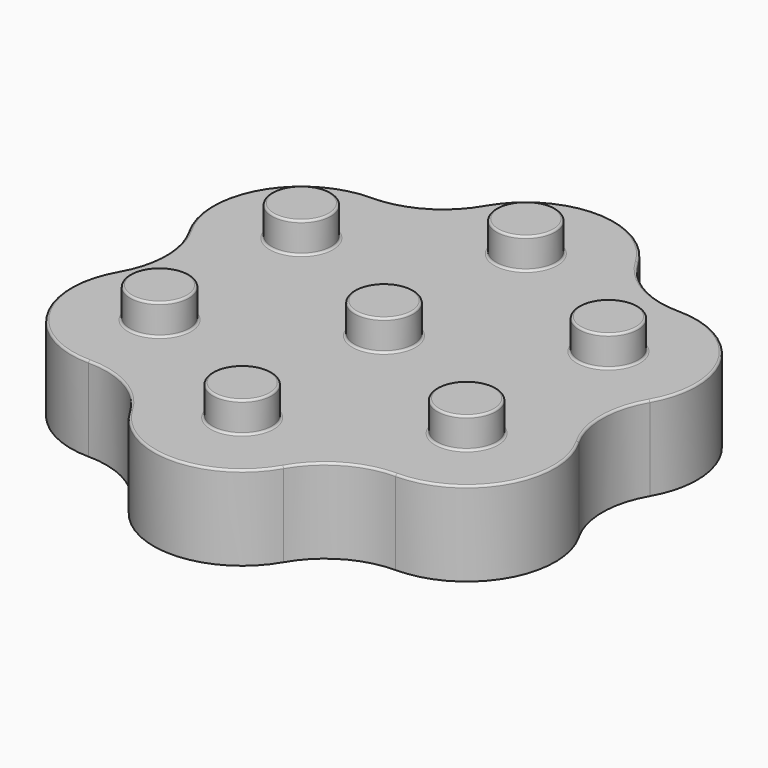
from build123d import *

# Parameters (mm, degrees)
F4_R     = 7.9
F5_DEPTH = 20
F6_DEPTH = 10
F7_R     = 7
F8_DEPTH = 7.3
F9_R     = 0.5


# Not quite as in the source:
# - a feature names something its author has since deleted; it is built from what else it names


with BuildPart() as f5:
    # F4 (on Top) → F5 (new body)
    with BuildSketch(Plane.XY):
        with BuildLine():
            ThreePointArc((18.1865334795, 10.5), (15.3730669589, 21), (18.1865334795, 31.5))
            ThreePointArc((18.1865334795, 31.5), (18.1865334795, 52.5), (0, 63))
            ThreePointArc((0, 63), (-10.5, 65.8134665205), (-18.1865334795, 73.5))
            ThreePointArc((-18.1865334795, 73.5), (-36.3730669589, 84), (-54.5596004384, 73.5))
            ThreePointArc((-54.5596004384, 73.5), (-62.2461339179, 65.8134665205), (-72.7461339179, 63))
            ThreePointArc((-72.7461339179, 63), (-90.9326673974, 52.5), (-90.9326673974, 31.5))
            ThreePointArc((-90.9326673974, 31.5), (-88.1192008768, 21), (-90.9326673974, 10.5))
            ThreePointArc((-90.9326673974, 10.5), (-90.9326673974, -10.5), (-72.7461339179, -21))
            ThreePointArc((-72.7461339179, -21), (-62.2461339179, -23.8134665205), (-54.5596004384, -31.5))
            ThreePointArc((-54.5596004384, -31.5), (-36.3730669589, -42), (-18.1865334795, -31.5))
            ThreePointArc((-18.1865334795, -31.5), (-10.5, -23.8134665205), (0, -21))
            ThreePointArc((0, -21), (18.1865334795, -10.5), (18.1865334795, 10.5))
        make_face()
        with Locations((-72.7461339179, 0)):
            Circle(F4_R, mode=Mode.SUBTRACT)
        with Locations((-36.3730669589, -21)):
            Circle(F4_R, mode=Mode.SUBTRACT)
        Circle(F4_R, mode=Mode.SUBTRACT)
        with Locations((-72.7461339179, 42)):
            Circle(F4_R, mode=Mode.SUBTRACT)
        with Locations((-36.3730669589, 21)):
            Circle(F4_R, mode=Mode.SUBTRACT)
        with Locations((0, 42)):
            Circle(F4_R, mode=Mode.SUBTRACT)
        with Locations((-36.3730669589, 63)):
            Circle(F4_R, mode=Mode.SUBTRACT)
        with Locations((0, 42)):
            Circle(F4_R)
        Circle(F4_R)
        with Locations((-36.3730669589, 21)):
            Circle(F4_R)
        with Locations((-36.3730669589, 63)):
            Circle(F4_R)
        with Locations((-72.7461339179, 42)):
            Circle(F4_R)
        with Locations((-72.7461339179, 0)):
            Circle(F4_R)
        with Locations((-36.3730669589, -21)):
            Circle(F4_R)
    extrude(amount=F5_DEPTH)

    # F4 (on Top) → F6 (cut)
    with BuildSketch(Plane.XY):
        with Locations((0, 42)):
            Circle(F4_R)
        Circle(F4_R)
        with Locations((-36.3730669589, 21)):
            Circle(F4_R)
        with Locations((-36.3730669589, 63)):
            Circle(F4_R)
        with Locations((-72.7461339179, 42)):
            Circle(F4_R)
        with Locations((-72.7461339179, 0)):
            Circle(F4_R)
        with Locations((-36.3730669589, -21)):
            Circle(F4_R)
    extrude(amount=F6_DEPTH, mode=Mode.SUBTRACT)

    # F7 (on face) → F8 (join)
    with BuildSketch(Plane.XY.offset(20)):
        Circle(F7_R)
        with Locations((0, 42)):
            Circle(F7_R)
        with Locations((-36.3730669589, 21)):
            Circle(F7_R)
        with Locations((-36.3730669589, 63)):
            Circle(F7_R)
        with Locations((-36.3730669589, -21)):
            Circle(F7_R)
        with Locations((-72.7461339179, 0)):
            Circle(F7_R)
        with Locations((-72.7461339179, 42)):
            Circle(F7_R)
    extrude(amount=F8_DEPTH)

    # F9
    f9_edges = [f5.edges().sort_by_distance(p)[0] for p in [
        (-7, 0, 27.3),
        (-7.9, 42, 0),
        (-7.9, 42, 10),
        (-7.9, 0, 0),
        (-7.9, 0, 10),
        (-7, 42, 27.3),
        (-7, 42, 20),
        (18.186533, 52.5, 20),
        (-43.373067, 21, 20),
        (-43.373067, 21, 27.3),
        (-28.473067, 21, 5),
        (-44.273067, 21, 0),
        (-44.273067, 21, 10),
        (-29.373067, 63, 23.65),
        (-43.373067, 63, 20),
        (-43.373067, 63, 27.3),
        (-28.473067, 63, 5),
        (-44.273067, 63, 0),
        (-44.273067, 63, 10),
        (-65.746134, 0, 23.65),
        (-79.746134, 0, 20),
        (-79.746134, 0, 27.3),
        (-29.373067, -21, 23.65),
        (-43.373067, -21, 20),
        (-43.373067, -21, 27.3),
        (-65.746134, 42, 23.65),
        (-79.746134, 42, 20),
        (-79.746134, 42, 27.3),
        (-64.846134, 42, 5),
        (-80.646134, 42, 0),
        (-80.646134, 42, 10),
        (-64.846134, 0, 5),
        (-80.646134, 0, 0),
        (-80.646134, 0, 10),
        (-28.473067, -21, 5),
        (-44.273067, -21, 0),
        (-44.273067, -21, 10),
        (-7, 0, 20),
    ]]
    fillet(f9_edges, radius=F9_R)


solid = f5.part
